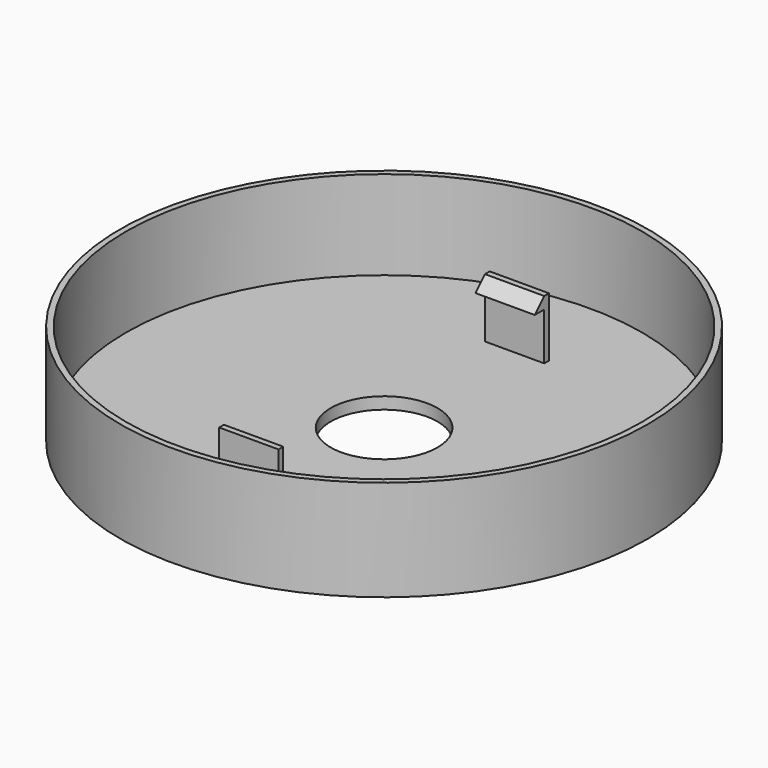
from build123d import *

# Parameters (mm, degrees)
F0_R      = 44.5
F1_DEPTH  = 2
F2_R      = 44.5
F2_R_2    = 43.5
F3_DEPTH  = 15
F4_R      = 9
F5_DEPTH  = 25
F7_W      = 10
F7_H      = 1
F8_DEPTH  = 10
F10_W     = 10
F10_H     = 2
F11_DEPTH = 2
F12_SIZE  = 1.99999


# Not quite as in the source:
# - a fillet or chamfer is up to 0.001 mm smaller than in the source, because OpenCascade refuses the exact size


with BuildPart() as f1:
    # F0 (on Top) → F1 (new body)
    with BuildSketch(Plane.XY):
        Circle(F0_R)
    extrude(amount=F1_DEPTH)

    # F2 (on face) → F3 (join)
    with BuildSketch(Plane.XY.offset(2)):
        Circle(F2_R)
        Circle(F2_R_2, mode=Mode.SUBTRACT)
    extrude(amount=F3_DEPTH)

    # F4 (on face) → F5 (cut)
    with BuildSketch(Plane.XY.offset(2)):
        Circle(F4_R)
    extrude(amount=-F5_DEPTH, mode=Mode.SUBTRACT)

    # F7 (on face) → F8 (join)
    with BuildSketch(Plane.XY.offset(2)):
        with Locations((0, 28)):
            Rectangle(F7_W, F7_H)
        with Locations((0, -28)):
            Rectangle(F7_W, F7_H)
    extrude(amount=F8_DEPTH)

    # F10 (on face) → F11 (join)
    with BuildSketch(Plane.XZ.offset(-27.5)):
        with Locations((0, 11)):
            Rectangle(F10_W, F10_H)
    extrude(amount=F11_DEPTH)

    # F12 (size 2 in the source; OpenCascade refuses exactly that, so slightly less here)
    f12_edges = [f1.edges().sort_by_distance(p)[0] for p in [
        (0, 25.5, 12),
    ]]
    chamfer(f12_edges, length=F12_SIZE)


solid = f1.part
